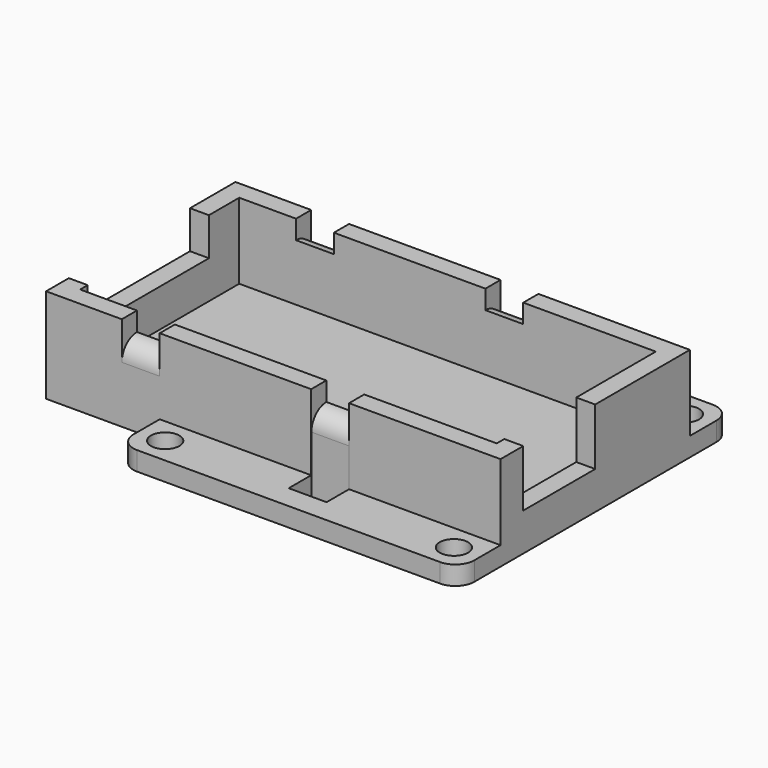
from build123d import *

# Parameters (mm, degrees)
F1_DEPTH     = 2
F2_R         = 2
F3_D         = 3
F6_W         = 2
F6_H         = 9.5
F7_DEPTH     = 2
F6_W_2       = 4
F6_H_2       = 2
F6_H_3       = 1.9668334348
F8_DEPTH     = 8
F6_W_3       = 16
F9_DEPTH     = 10
F10_T1_DEPTH = 4
F10_T3_DEPTH = 4
F11_DEPTH    = 4
F6_H_4       = 16
F12_DEPTH    = 6


# Not quite as in the source:
# - a fillet or chamfer that OpenCascade refuses, or shapes differently, is made with other operations: its cross-section is extruded or revolved along the edge and cut away or added
# - a feature names something its author has since deleted; it is built from what else it names


with BuildPart() as f1:
    # F0 (on Top) → F1 (new body)
    with BuildSketch(Plane.XY):
        Polygon((-19.8978664808, -19.9668334348), (-1.8978664808, -19.9668334348), (-1.8978664808, -17.4668334348), (-3.8978664808, -17.4668334348), (-3.8978664808, -14.4668334348), (-1.8978664808, -14.4668334348), (-1.8978664808, -1.9668334348), (-19.8978664808, -1.9668334348), align=None)
    extrude(amount=F1_DEPTH)

    # F2
    f2_edges = [f1.edges().sort_by_distance(p)[0] for p in [
        (-19.897866, -19.966833, 1),
    ]]
    fillet(f2_edges, radius=F2_R)

    # F3 (through all)
    with Locations(Plane(origin=(0, 0, 0), x_dir=(1, 0, 0), z_dir=(0, 0, -1))):
        with Locations((-17.1478664808, 17.2168334348)):
            Hole(F3_D / 2)

    # F4: F1 across face


with BuildPart() as f1_1:
    add(f1.part)
    add(f1.part.mirror(Plane(origin=(-1.8978664808, -8.2168334348, 1), x_dir=(0, 1, 0), z_dir=(1, 0, 0))))

    # F5: F1 across face


with BuildPart() as f1_2:
    add(f1_1.part)
    add(f1_1.part.mirror(Plane(origin=(-1.8978664808, -1.9668334348, 1), x_dir=(-1, 0, 0), z_dir=(0, 1, 0))))

    # F6 (on face) → F7 (join)
    with BuildSketch(Plane(origin=(0, 0, 0), x_dir=(1, 0, 0), z_dir=(0, 0, -1))):
        Polygon((-29.8978664808, -8.5), (-23.8978664808, -8.5), (-19.8978664808, -8.5), (-19.8978664808, 12.5), (-23.8978664808, 12.5), (-29.8978664808, 12.5), (-29.8978664808, 11.5), (-29.8978664808, -4.5), align=None)
        with Locations((15.1021335192, 6.75)):
            Rectangle(F6_W, F6_H)
        Polygon((-19.8978664808, 12.5), (-19.8978664808, -8.5), (-3.8978664808, -8.5), (0.1021335192, -8.5), (14.1021335192, -8.5), (14.1021335192, 2), (14.1021335192, 11.5), (14.1021335192, 12.5), (0.1021335192, 12.5), (-3.8978664808, 12.5), align=None)
    extrude(amount=-F7_DEPTH)

    # F6 (on face) → F8 (join)
    with BuildSketch(Plane(origin=(0, 0, 0), x_dir=(1, 0, 0), z_dir=(0, 0, -1))):
        with Locations((-1.8978664808, -9.5)):
            Rectangle(F6_W_2, F6_H_2)
        with Locations((-1.8978664808, 13.4834167174)):
            Rectangle(F6_W_2, F6_H_3)
        with Locations((-21.8978664808, 13.5)):
            Rectangle(F6_W_2, F6_H_2)
        with Locations((-21.8978664808, -9.5)):
            Rectangle(F6_W_2, F6_H_2)
    extrude(amount=-F8_DEPTH)

    # F6 (on face) → F9 (join)
    with BuildSketch(Plane(origin=(0, 0, 0), x_dir=(1, 0, 0), z_dir=(0, 0, -1))):
        Polygon((-31.8978664808, -10.5), (-23.8978664808, -10.5), (-23.8978664808, -8.5), (-29.8978664808, -8.5), (-29.8978664808, -4.5), (-31.8978664808, -4.5), align=None)
        Polygon((0.1021335192, -8.5), (0.1021335192, -10.5), (16.1021335192, -10.5), (16.1021335192, 2), (14.1021335192, 2), (14.1021335192, -8.5), align=None)
        Polygon((0.1021335192, 14.4668334348), (0.1021335192, 12.5), (14.1021335192, 12.5), (14.1021335192, 11.5), (16.1021335192, 11.5), (16.1021335192, 14.5), (0.1021335192, 14.5), align=None)
        Polygon((-19.8978664808, 14.5), (-19.8978664808, 12.5), (-3.8978664808, 12.5), (-3.8978664808, 14.4668334348), (-3.8978664808, 14.5), align=None)
        Polygon((-31.8978664808, 14.5), (-31.8978664808, 11.5), (-29.8978664808, 11.5), (-29.8978664808, 12.5), (-23.8978664808, 12.5), (-23.8978664808, 14.5), align=None)
        with Locations((-11.8978664808, -9.5)):
            Rectangle(F6_W_3, F6_H_2)
    extrude(amount=-F9_DEPTH)

    # F10: fillet of radius 2 on 4 edges, made by hand

    # F10_s2 → F10_t1 (cut)
    with BuildSketch(Plane.YZ.offset(-3.8978664808)):
        with BuildLine():
            ThreePointArc((-14.4668334348, 6), (-13.8810469972, 7.4142135624), (-12.4668334348, 8))
            Line((-12.4668334348, 8), (-14.4668334348, 8))
            Line((-14.4668334348, 8), (-14.4668334348, 6))
        make_face()
        with BuildLine():
            ThreePointArc((8.5, 8), (9.9142135624, 7.4142135624), (10.5, 6))
            Line((10.5, 6), (10.5, 8))
            Line((10.5, 8), (8.5, 8))
        make_face()
    extrude(amount=F10_T1_DEPTH, mode=Mode.SUBTRACT)

    # F10_s4 → F10_t3 (cut)
    with BuildSketch(Plane.YZ.offset(-23.8978664808)):
        with BuildLine():
            ThreePointArc((8.5, 8), (9.9142135624, 7.4142135624), (10.5, 6))
            Line((10.5, 6), (10.5, 8))
            Line((10.5, 8), (8.5, 8))
        make_face()
        with BuildLine():
            ThreePointArc((-14.5, 6), (-13.9142135624, 7.4142135624), (-12.5, 8))
            Line((-12.5, 8), (-14.5, 8))
            Line((-14.5, 8), (-14.5, 6))
        make_face()
    extrude(amount=F10_T3_DEPTH, mode=Mode.SUBTRACT)

    # F6 (on face) → F11 (join)
    with BuildSketch(Plane(origin=(0, 0, 0), x_dir=(1, 0, 0), z_dir=(0, 0, -1))):
        with Locations((15.1021335192, 6.75)):
            Rectangle(F6_W, F6_H)
    extrude(amount=-F11_DEPTH)

    # F6 (on face) → F12 (join)
    with BuildSketch(Plane(origin=(0, 0, 0), x_dir=(1, 0, 0), z_dir=(0, 0, -1))):
        with Locations((-30.8978664808, 3.5)):
            Rectangle(F6_W, F6_H_4)
    extrude(amount=-F12_DEPTH)


solid = f1_2.part
